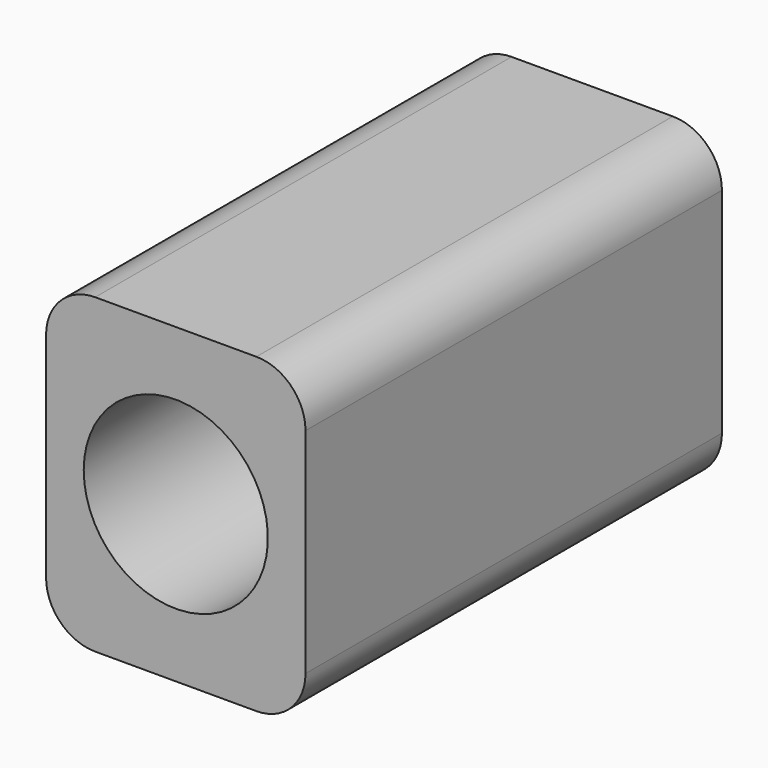
from build123d import *

# Parameters (mm, degrees)
F0_W     = 26.8379747868
F0_H     = 32.2756916285
F1_DEPTH = 53.848
F2_R     = 10.4478277996
F3_DEPTH = 43.688
F7_D     = 19.05
F7_DEPTH = 44.45
F7_TIP   = 5.7231973962
F8_R     = 5.08


# Not quite as in the source:
# - the program builds the solid bodies; features that only make, move or delete a surface that nothing else refers to are left out


with BuildPart() as f1:
    # F0 (on Front) → F1 (new body)
    with BuildSketch(Plane.XZ):
        with Locations((13.4189873934, 16.1378458142)):
            Rectangle(F0_W, F0_H)
    extrude(amount=F1_DEPTH)

    # F2 (on face) → F3 (join)
    with BuildSketch(Plane.XZ.offset(53.848)):
        with Locations((11.908470653, 14.5087121055)):
            Circle(F2_R)
    extrude(amount=-F3_DEPTH)

    # F7
    with Locations(Plane.XZ.offset(53.848)):
        with Locations((13.4189873934, 16.1378458142)):
            Hole(F7_D / 2, depth=F7_DEPTH)
            with Locations((0, 0, -(F7_DEPTH + F7_TIP / 2))):  # 118° drill point
                Cone(0, F7_D / 2, F7_TIP, mode=Mode.SUBTRACT)

    # F8
    f8_edges = [f1.edges().sort_by_distance(p)[0] for p in [
        (0, -26.924, 32.275692),
        (26.837975, -26.924, 32.275692),
        (26.837975, -26.924, 0),
        (0, -26.924, 0),
    ]]
    fillet(f8_edges, radius=F8_R)


solid = f1.part
